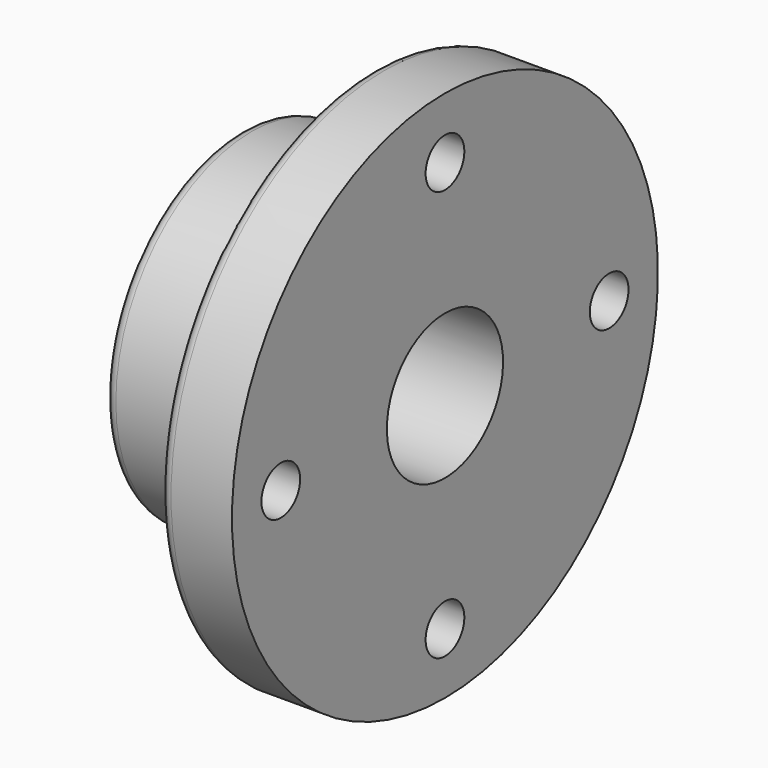
from build123d import *

# Parameters (mm, degrees)
F2_R     = 6.35
F3_DEPTH = 53.849
F4_R     = 3.04799
F5_R     = 3.048


# Not quite as in the source:
# - a fillet or chamfer is up to 0.001 mm smaller than in the source, because OpenCascade refuses the exact size


with BuildPart() as f1:
    # F0 (on Front) → F1 (revolve)
    with BuildSketch(Plane.XZ):
        Polygon((0, 44.45), (0, 19.05), (53.848, 19.05), (53.848, 69.85), (34.798, 69.85), (34.798, 44.45), align=None)
    revolve(axis=Axis((45.7144924702, 0, 0), (1, 0, 0)))

    # F2 (on Right) → F3 (cut, through all)
    with BuildSketch(Plane.YZ):
        with Locations((0, 53.848)):
            Circle(F2_R)
        with Locations((53.848, 0)):
            Circle(F2_R)
        with Locations((-53.848, 0)):
            Circle(F2_R)
        with Locations((0, -53.848)):
            Circle(F2_R)
    extrude(amount=F3_DEPTH, mode=Mode.SUBTRACT)

    # F4 (radius 3.048 in the source; OpenCascade refuses exactly that, so slightly less here)
    f4_edges = [f1.edges().sort_by_distance(p)[0] for p in [
        (34.798, 0, -44.45),
    ]]
    fillet(f4_edges, radius=F4_R)

    # F5
    f5_edges = [f1.edges().sort_by_distance(p)[0] for p in [
        (0, 0, -44.45),
        (34.798, 0, -69.85),
    ]]
    fillet(f5_edges, radius=F5_R)


solid = f1.part
